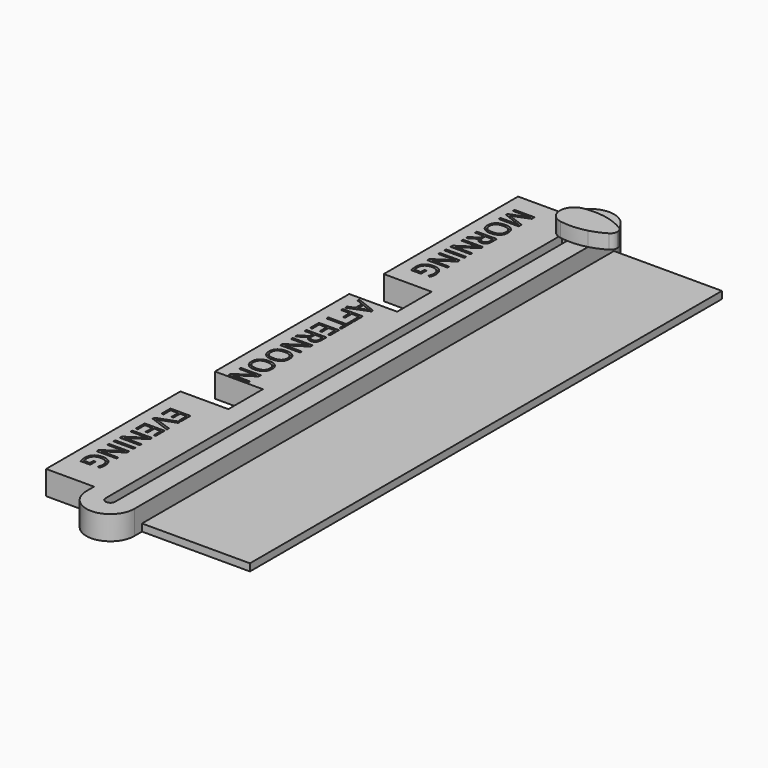
from build123d import *

# Parameters (mm, degrees)
F1_DEPTH      = 10
F2_W          = 20
F2_H          = 70
F3_DEPTH      = 10
F5_DEPTH      = 6
F6_W          = 45
F6_H          = 246
F7_DEPTH      = 3
F10_DEPTH     = 25
F11_W         = 2.6455906918
F11_H         = 9.9265053868
F12_DEPTH     = 3
F13_TEXT_SIZE = 11.6791625845
F14_DEPTH     = 1
F16_DEPTH     = 2.5


# Not quite as in the source:
# - Text() gives the source's letters only with a copy of the font that has no kerning and outlines rounded to 1/6400 em; it was checked with that copy


with BuildPart() as f1:
    # F0 (on Top) → F1 (new body)
    with BuildSketch(Plane.XY):
        with BuildLine():
            ThreePointArc((10, 125), (0, 135), (-10, 125))
            Line((-10, 125), (-10, -125))
            ThreePointArc((-10, -125), (0, -135), (10, -125))
            Line((10, -125), (10, 125))
        make_face()
    extrude(amount=-F1_DEPTH)

    # F2 (on face) → F3 (join, through all)
    with BuildSketch(Plane.XY):
        with Locations((-20, 90)):
            Rectangle(F2_W, F2_H)
        with Locations((-20, 2)):
            Rectangle(F2_W, F2_H)
        with Locations((-20, -86)):
            Rectangle(F2_W, F2_H)
    extrude(amount=-F3_DEPTH)

    # F6 (on face) → F7 (join)
    with BuildSketch(Plane(origin=(0, 0, -10), x_dir=(1, 0, 0), z_dir=(0, 0, -1))):
        with Locations((32.5, -2)):
            Rectangle(F6_W, F6_H)
    extrude(amount=-F7_DEPTH)

    # F9 (on face) → F10 (cut)
    with BuildSketch(Plane.XY):
        with BuildLine():
            ThreePointArc((2, 125), (0, 127), (-2, 125))
            Line((-2, 125), (-2, -125))
            ThreePointArc((-2, -125), (0, -127), (2, -125))
            Line((2, -125), (2, 125))
        make_face()
    extrude(amount=-F10_DEPTH, mode=Mode.SUBTRACT)

    # F13 (on face) → F14 (cut)
    with BuildSketch(Plane.XY):
        with Locations(Location((-25, 118.0692411191), (0, 0, -90))):
            Text('MORNING', F13_TEXT_SIZE, font='Open Sans', text_align=(TextAlign.LEFT, TextAlign.BOTTOM))
        with Locations(Location((-25, 36.0056021831), (0, 0, -90))):
            Text('AFTERNOON', F13_TEXT_SIZE, font='Open Sans', text_align=(TextAlign.LEFT, TextAlign.BOTTOM))
        with Locations(Location((-25, -61.2652272415), (0, 0, -90))):
            Text('EVENING', F13_TEXT_SIZE, font='Open Sans', text_align=(TextAlign.LEFT, TextAlign.BOTTOM))
    extrude(amount=-F14_DEPTH, mode=Mode.SUBTRACT)

    # F15 (on face) → F16 (join)
    with BuildSketch(Plane(origin=(0, 0, -10), x_dir=(1, 0, 0), z_dir=(0, 0, -1))):
        with BuildLine():
            ThreePointArc((-2, -125), (0, -127), (2, -125))
            Line((2, -125), (2, 125))
            ThreePointArc((2, 125), (0, 127), (-2, 125))
            Line((-2, 125), (-2, -125))
        make_face()
    extrude(amount=-F16_DEPTH)


with BuildPart() as f5:
    # F4 (on face) → F5 (new body)
    with BuildSketch(Plane.XY):
        with BuildLine():
            Line((0, 116.8112903833), (0, 122.8112903833))
            ThreePointArc((0, 122.8112903833), (-0.500806832, 122.7903532294), (-0.9981185075, 122.727687889))
            ThreePointArc((-0.9981185075, 122.727687889), (-6, 116.8112903833), (-0.9981185075, 110.8948928777))
            ThreePointArc((-0.9981185075, 110.8948928777), (3.8737119766, 112.2293305928), (6, 116.8112903833))
            Line((6, 116.8112903833), (0, 116.8112903833))
        make_face()
        with BuildLine():
            ThreePointArc((6, 116.8112903833), (4.2426406871, 121.0539310705), (0, 122.8112903833))
            Line((0, 122.8112903833), (0, 116.8112903833))
            Line((0, 116.8112903833), (6, 116.8112903833))
        make_face()
        with BuildLine():
            ThreePointArc((10, 122.1864309392), (5.0340054601, 123.0243674318), (0, 122.875947879))
            Line((0, 122.875947879), (0, 122.8112903833))
            ThreePointArc((0, 122.8112903833), (4.2426406871, 121.0539310705), (6, 116.8112903833))
            Line((6, 116.8112903833), (10, 116.8112903833))
            Line((10, 116.8112903833), (10, 122.1864309392))
        make_face()
        with BuildLine():
            ThreePointArc((16.5535088719, 119.3777295868), (13.3748112683, 121.0108750831), (10, 122.1864309392))
            Line((10, 122.1864309392), (10, 116.8112903833))
            Line((10, 116.8112903833), (12, 116.8112903833))
            ThreePointArc((12, 116.8112903833), (13.526997389, 119.4247676279), (16.5535088719, 119.3777295868))
        make_face()
        with BuildLine():
            ThreePointArc((18, 116.8112903833), (17.6134772446, 118.2842929944), (16.5535088719, 119.3777295868))
            ThreePointArc((16.5535088719, 119.3777295868), (13.526997389, 119.4247676279), (12, 116.8112903833))
            ThreePointArc((12, 116.8112903833), (13.526997389, 114.1978131388), (16.5535088719, 114.2448511799))
            ThreePointArc((16.5535088719, 114.2448511799), (17.6134772446, 115.3382877723), (18, 116.8112903833))
        make_face()
        with BuildLine():
            Line((12, 116.8112903833), (10, 116.8112903833))
            Line((10, 116.8112903833), (10, 111.4361498275))
            ThreePointArc((10, 111.4361498275), (13.3748112683, 112.6117056835), (16.5535088719, 114.2448511799))
            ThreePointArc((16.5535088719, 114.2448511799), (13.526997389, 114.1978131388), (12, 116.8112903833))
        make_face()
        with BuildLine():
            Line((10, 116.8112903833), (6, 116.8112903833))
            ThreePointArc((6, 116.8112903833), (3.8737119766, 112.2293305928), (-0.9981185075, 110.8948928777))
            ThreePointArc((-0.9981185075, 110.8948928777), (4.5303244091, 110.5684574145), (10, 111.4361498275))
            Line((10, 111.4361498275), (10, 116.8112903833))
        make_face()
    extrude(amount=F5_DEPTH)

    # F11 (on face) → F12 (join)
    with BuildSketch(Plane.XY):
        with Locations((-0.2317862236, 117.2381155193)):
            Rectangle(F11_W, F11_H)
    extrude(amount=-F12_DEPTH)


solid = Compound([f1.part, f5.part])
